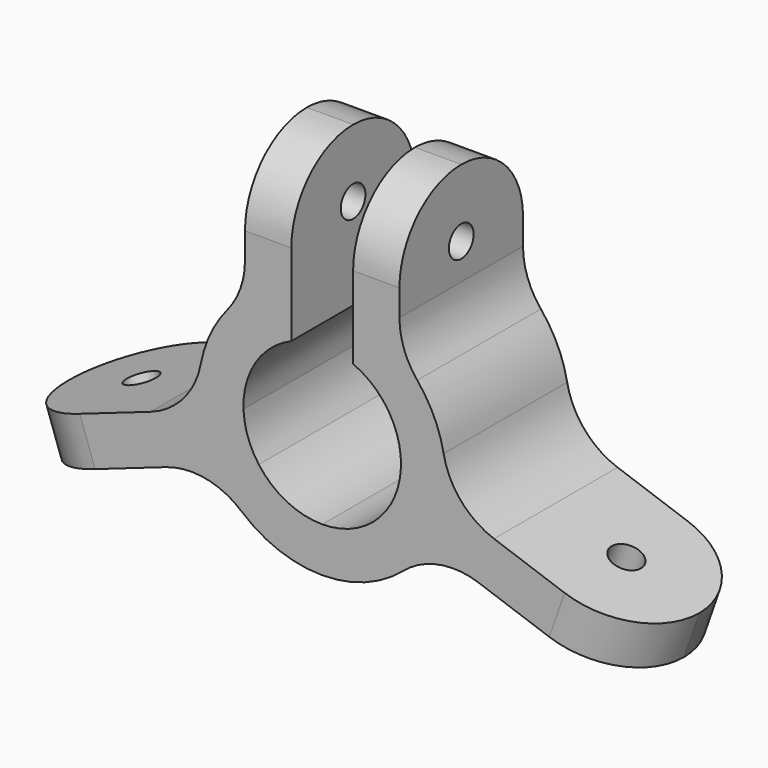
from build123d import *

# Parameters (mm, degrees)
F1_DEPTH = 5
F2_R     = 1
F3_DEPTH = 25
F4_R     = 1
F5_DEPTH = 25
F6_R     = 4.99999
F7_R     = 5


# Not quite as in the source:
# - a fillet or chamfer is up to 0.001 mm smaller than in the source, because OpenCascade refuses the exact size
# - a feature names something its author has since deleted; it is built from what else it names


with BuildPart() as f1:
    # F0 (on Front) → F1 (new body, symmetric)
    with BuildSketch(Plane.XZ):
        with BuildLine():
            ThreePointArc((4.105083276, -3.0262668912), (2.2995694004, -4.5521402189), (0, -5.1))
            Line((0, -5.1), (0, -8))
            ThreePointArc((0, -8), (3.9939571451, -6.9316885622), (6.9212167652, -4.0120765807))
            Line((6.9212167652, -4.0120765807), (4.105083276, -3.0262668912))
        make_face()
        with BuildLine():
            ThreePointArc((5.0962805256, -0.1947429178), (4.8135907549, -1.6850353244), (4.105083276, -3.0262668912))
            Line((4.105083276, -3.0262668912), (6.9212167652, -4.0120765807))
            ThreePointArc((6.9212167652, -4.0120765807), (7.5507305959, -2.6431926657), (7.9124140148, -1.1805526072))
            Line((7.9124140148, -1.1805526072), (5.0962805256, -0.1947429178))
        make_face()
        with BuildLine():
            ThreePointArc((2, 4.6914816423), (4.3079109714, 2.7298174046), (5.0962805256, -0.1947429178))
            Line((5.0962805256, -0.1947429178), (7.9124140148, -1.1805526072))
            ThreePointArc((7.9124140148, -1.1805526072), (7.4476378384, 2.9210769638), (5, 6.2449979984))
            ThreePointArc((5, 6.2449979984), (3.5795567819, 7.1544932207), (2, 7.7459666924))
            Line((2, 7.7459666924), (2, 4.6914816423))
        make_face()
        with BuildLine():
            ThreePointArc((7.9124140148, -1.1805526072), (7.5507305959, -2.6431926657), (6.9212167652, -4.0120765807))
            Line((6.9212167652, -4.0120765807), (19.4194533219, -8.3871826424))
            Line((19.4194533219, -8.3871826424), (20.4106505716, -5.555658669))
            Line((20.4106505716, -5.555658669), (7.9124140148, -1.1805526072))
        make_face()
        with BuildLine():
            Line((2, 15), (2, 7.7459666924))
            ThreePointArc((2, 7.7459666924), (3.5795567819, 7.1544932207), (5, 6.2449979984))
            Line((5, 6.2449979984), (5, 15))
            Line((5, 15), (2, 15))
        make_face()
    extrude(amount=F1_DEPTH, both=True)

    # F2 (on face) → F3 (cut)
    with BuildSketch(Plane(origin=(0.4955986248, 0, 1.4157619867), x_dir=(0.9438413245, 0, -0.3303990832), z_dir=(0.3303990832, 0, 0.9438413245))):
        with Locations((16.1, 0)):
            Circle(F2_R)
    extrude(amount=-F3_DEPTH, mode=Mode.SUBTRACT)

    # F4 (on face) → F5 (cut)
    with BuildSketch(Plane.YZ.offset(5)):
        with Locations((0, 10.6224989992)):
            Circle(F4_R)
    extrude(amount=-F5_DEPTH, mode=Mode.SUBTRACT)

    # F6 (radius 5 in the source; OpenCascade refuses exactly that, so slightly less here)
    f6_edges = [f1.edges().sort_by_distance(p)[0] for p in [
        (19.915052, 5, -6.971421),
        (19.915052, -5, -6.971421),
        (3.5, -5, 15),
        (3.5, 5, 15),
    ]]
    fillet(f6_edges, radius=F6_R)

    # F7
    f7_edges = [f1.edges().sort_by_distance(p)[0] for p in [
        (5, 0, 6.244998),
        (7.912414, 0, -1.180553),
        (6.921217, 0, -4.012077),
    ]]
    fillet(f7_edges, radius=F7_R)

    # F8: F1 across plane


with BuildPart() as f1_1:
    add(f1.part)
    add(f1.part.mirror(Plane.YZ))


solid = f1_1.part
